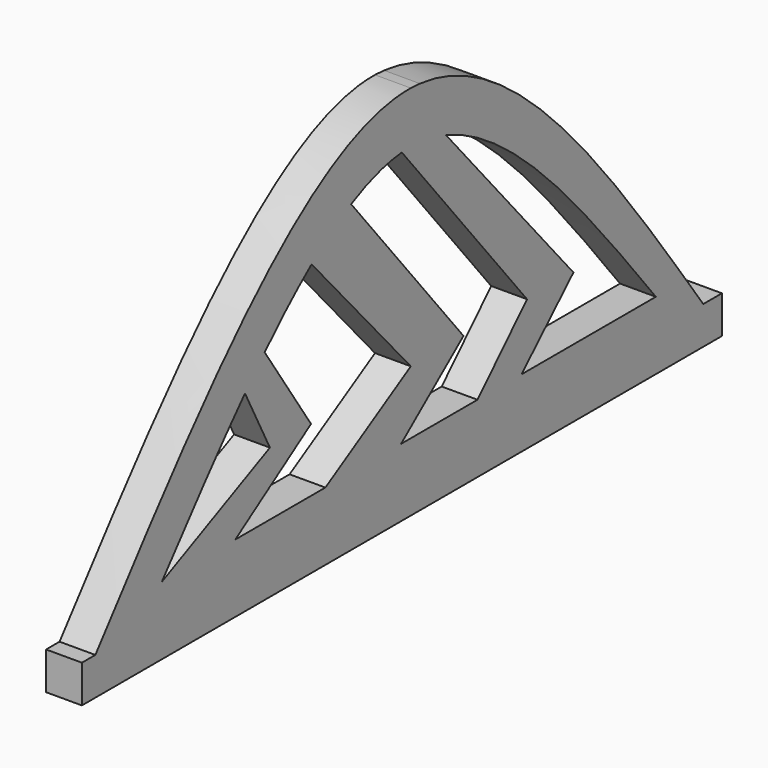
from build123d import *

# Parameters (mm, degrees)
F1_DEPTH = 7.62


with BuildPart() as f1:
    # F0 (on Right) → F1 (new body)
    with BuildSketch(Plane.YZ):
        with BuildLine():
            Line((-83.8999077678, 0), (-76.0438218713, 0))
            Line((-76.0438218713, 0), (-68.3361637849, 0))
            Line((-68.3361637849, 0), (-65.6663442796, 0))
            Line((-65.6663442796, 0), (-59.0906857838, 0))
            Line((-59.0906857838, 0), (-56.6208846061, 0))
            Line((-56.6208846061, 0), (-50.1111261547, 0))
            Line((-50.1111261547, 0), (-47.2127646201, 0))
            Line((-47.2127646201, 0), (-40.9584082663, 0))
            Line((-40.9584082663, 0), (-38.0600504577, 0))
            Line((-38.0600504577, 0), (-31.6531471908, 0))
            Line((-31.6531471908, 0), (-28.9073325694, 0))
            Line((-28.9073325694, 0), (-22.5004293025, 0))
            Line((-22.5004293025, 0), (-19.9071597308, 0))
            Line((-19.9071597308, 0), (-13.4495065357, 0))
            Line((-13.4495065357, 0), (-10.754442774, 0))
            Line((-10.754442774, 0), (-4.1949953884, 0))
            Line((-4.1949953884, 0), (-1.6017258168, 0))
            Line((-1.6017258168, 0), (4.8051769845, 0))
            Line((4.8051769845, 0), (7.3984456249, 0))
            Line((7.3984456249, 0), (13.8053493574, 0))
            Line((13.8053493574, 0), (16.7037080973, 0))
            Line((16.7037080973, 0), (23.1106095016, 0))
            Line((23.1106095016, 0), (25.7038809359, 0))
            Line((25.7038809359, 0), (32.1107842028, 0))
            Line((32.1107842028, 0), (34.5515049994, 0))
            Line((34.5515049994, 0), (40.958404541, 0))
            Line((40.958404541, 0), (43.7042228877, 0))
            Line((43.7042228877, 0), (50.1111261552, 0))
            Line((50.1111261552, 0), (52.7043938637, 0))
            Line((52.7043938637, 0), (59.263844043, 0))
            Line((59.263844043, 0), (61.8571154775, 0))
            Line((61.8571154775, 0), (72.8403702378, 0))
            Line((72.8403702378, 0), (77.7980908751, 0))
            add(Edge.make_bspline(
                [(2.4155534392, 71.935541455), (28.1982811761, 69.4119022605), (52.9981860256, 34.7059511303), (77.7980908751, 0)],
                knots=[0.5202204491, 0.5202204491, 0.5202204491, 0.5202204491, 1, 1, 1, 1], degree=3))
            add(Edge.make_bspline(
                [(2.4155534392, 71.935541455), (23.457256807, 69.5741418959), (44.3202320999, 38.0280369375), (65.1832073927, 6.4819319791)],
                knots=[0.5194057291, 0.5194057291, 0.5194057291, 0.5194057291, 1, 1, 1, 1], degree=3))
            Line((65.1832073927, 6.4819319791), (29.4485222548, 6.4819319791))
            Line((29.4485222548, 6.4819319791), (17.7436252383, 6.4819319791))
            Line((17.7436252383, 6.4819319791), (-2.5848655496, 6.4819319791))
            Line((-2.5848655496, 6.4819319791), (-22.7159410715, 6.4819319791))
            Line((-22.7159410715, 6.4819319791), (-46.667508781, 6.4819319791))
            Line((-46.667508781, 6.4819319791), (-66.2550926208, 6.4819319791))
            add(Edge.make_bspline(
                [(-66.2550926208, 6.4819319791), (-44.7386888592, 38.3814174671), (-23.2222850975, 70.2809029552), (-1.8906832982, 72.0038712376)],
                knots=[0, 0, 0, 0, 0.4866401258, 0.4866401258, 0.4866401258, 0.4866401258], degree=3))
            add(Edge.make_bspline(
                [(-1.8906832982, 72.0038712376), (-1.2602925513, 72.0547883357), (-0.6300631821, 72.0793517198), (2.66e-08, 72.0767825841)],
                knots=[0.4866401258, 0.4866401258, 0.4866401258, 0.4866401258, 0.5010212977, 0.5010212977, 0.5010212977, 0.5010212977], degree=3))
            add(Edge.make_bspline(
                [(-83.8999077678, 0), (-55.5586168349, 36.2935873023), (-27.217325902, 72.5871746046), (0, 72.0767825842)],
                knots=[0, 0, 0, 0, 0.505255101, 0.505255101, 0.505255101, 0.505255101], degree=3))
        make_face()
        Polygon((-68.3361637849, 0), (-76.0438218713, 0), (-83.8999077678, 0), (-87.4847173691, 0), (-87.4847173691, -8.0094942823), (82.7558115125, -8.0094942823), (82.7558115125, 0), (77.7980908751, 0), (72.8403702378, 0), (61.8571154775, 0), (59.263844043, 0), (52.7043938637, 0), (50.1111261552, 0), (43.7042228877, 0), (40.958404541, 0), (34.5515049994, 0), (32.1107842028, 0), (25.7038809359, 0), (23.1106095016, 0), (16.7037080973, 0), (13.8053493574, 0), (7.3984456249, 0), (4.8051769845, 0), (-1.6017258168, 0), (-4.1949953884, 0), (-10.754442774, 0), (-13.4495065357, 0), (-19.9071597308, 0), (-22.5004293025, 0), (-28.9073325694, 0), (-31.6531471908, 0), (-38.0600504577, 0), (-40.9584082663, 0), (-47.2127646201, 0), (-50.1111261547, 0), (-56.6208846061, 0), (-59.0906857838, 0), (-65.6663442796, 0), align=None)
        with BuildLine():
            add(Edge.make_bspline(
                [(0, 72.0767825842), (0.8061606012, 72.0616650837), (1.6113351386, 72.0142591471), (2.4155534392, 71.935541455)],
                knots=[0.505255101, 0.505255101, 0.505255101, 0.505255101, 0.5202204491, 0.5202204491, 0.5202204491, 0.5202204491], degree=3))
            add(Edge.make_bspline(
                [(-1.8906832982, 72.0038712376), (-1.2602925513, 72.0547883357), (-0.6300631821, 72.0793517198), (2.66e-08, 72.0767825841)],
                knots=[0.4866401258, 0.4866401258, 0.4866401258, 0.4866401258, 0.5010212977, 0.5010212977, 0.5010212977, 0.5010212977], degree=3))
            add(Edge.make_bspline(
                [(-66.2550926208, 6.4819319791), (-44.7386888592, 38.3814174671), (-23.2222850975, 70.2809029552), (-1.8906832982, 72.0038712376)],
                knots=[0, 0, 0, 0, 0.4866401258, 0.4866401258, 0.4866401258, 0.4866401258], degree=3))
            add(Edge.make_bspline(
                [(-66.2550926208, 6.4819319791), (-58.870002531, 15.6014280008), (-51.4849124411, 24.7209240225), (-44.1068523116, 32.8232360474)],
                knots=[0, 0, 0, 0, 0.1671216862, 0.1671216862, 0.1671216862, 0.1671216862], degree=3))
            add(Edge.make_bspline(
                [(-44.1068523116, 32.8232360474), (-42.3619029204, 34.7394747588), (-40.6173467479, 36.5988175914), (-38.8732767924, 38.3878083756)],
                knots=[0.1671216862, 0.1671216862, 0.1671216862, 0.1671216862, 0.2066468296, 0.2066468296, 0.2066468296, 0.2066468296], degree=3))
            add(Edge.make_bspline(
                [(-38.8732767924, 38.3878083756), (-34.7114395699, 42.6568392208), (-30.5523710257, 46.5252625196), (-26.3973348433, 49.8102324575)],
                knots=[0.2066468296, 0.2066468296, 0.2066468296, 0.2066468296, 0.3009648428, 0.3009648428, 0.3009648428, 0.3009648428], degree=3))
            add(Edge.make_bspline(
                [(-26.3973348433, 49.8102324575), (-22.8832827761, 52.5884406113), (-19.3721149148, 54.9493251989), (-15.8645956908, 56.7822785692)],
                knots=[0.3009648428, 0.3009648428, 0.3009648428, 0.3009648428, 0.3807327183, 0.3807327183, 0.3807327183, 0.3807327183], degree=3))
            add(Edge.make_bspline(
                [(-15.8645956908, 56.7822785692), (-11.3638797078, 59.1342549956), (-6.8691712251, 60.6169899499), (-2.3820852822, 60.9967989829)],
                knots=[0.3807327183, 0.3807327183, 0.3807327183, 0.3807327183, 0.4830878387, 0.4830878387, 0.4830878387, 0.4830878387], degree=3))
            add(Edge.make_bspline(
                [(-2.3820852822, 60.9967989829), (-1.5878150287, 61.0640299254), (2.3324808206, 61.2253407539), (6.2467363494, 60.5126612784), (9.3648919901, 59.4680160873)],
                knots=[0.4830878387, 0.4830878387, 0.4830878387, 0.4830878387, 0.5012059734, 0.5725407835, 0.5725407835, 0.5725407835, 0.5725407835], degree=3))
            add(Edge.make_bspline(
                [(9.3648919901, 59.4680160873), (28.0498000323, 53.2081940706), (46.6165037125, 29.8450630249), (65.1832073927, 6.4819319791)],
                knots=[0.5725407835, 0.5725407835, 0.5725407835, 0.5725407835, 1, 1, 1, 1], degree=3))
            add(Edge.make_bspline(
                [(2.4155534392, 71.935541455), (23.457256807, 69.5741418959), (44.3202320999, 38.0280369375), (65.1832073927, 6.4819319791)],
                knots=[0.5194057291, 0.5194057291, 0.5194057291, 0.5194057291, 1, 1, 1, 1], degree=3))
        make_face()
        with BuildLine():
            Line((-37.4757476613, 19.9564792332), (-66.2550926208, 6.4819319791))
            Line((-66.2550926208, 6.4819319791), (-46.667508781, 6.4819319791))
            Line((-46.667508781, 6.4819319791), (-26.5364367513, 19.9564792332))
            Line((-26.5364367513, 19.9564792332), (-38.8732767924, 38.3878083756))
            add(Edge.make_bspline(
                [(-44.1068523116, 32.8232360474), (-42.3619029204, 34.7394747588), (-40.6173467479, 36.5988175914), (-38.8732767924, 38.3878083756)],
                knots=[0.1671216862, 0.1671216862, 0.1671216862, 0.1671216862, 0.2066468296, 0.2066468296, 0.2066468296, 0.2066468296], degree=3))
            Line((-44.1068523116, 32.8232360474), (-37.4757476613, 19.9564792332))
        make_face()
        with BuildLine():
            Line((17.7436252383, 6.4819319791), (29.4485222548, 6.4819319791))
            Line((29.4485222548, 6.4819319791), (43.261088431, 19.9564792332))
            Line((43.261088431, 19.9564792332), (9.3648919901, 59.4680160873))
            add(Edge.make_bspline(
                [(-2.3820852822, 60.9967989829), (-1.5878150287, 61.0640299254), (2.3324808206, 61.2253407539), (6.2467363494, 60.5126612784), (9.3648919901, 59.4680160873)],
                knots=[0.4830878387, 0.4830878387, 0.4830878387, 0.4830878387, 0.5012059734, 0.5725407835, 0.5725407835, 0.5725407835, 0.5725407835], degree=3))
            Line((-2.3820852822, 60.9967989829), (30.9179425241, 19.9564792332))
            Line((30.9179425241, 19.9564792332), (17.7436252383, 6.4819319791))
        make_face()
        with BuildLine():
            Line((0, 19.9564792332), (-22.7159410715, 6.4819319791))
            Line((-22.7159410715, 6.4819319791), (-2.5848655496, 6.4819319791))
            Line((-2.5848655496, 6.4819319791), (14.0195973219, 19.9564792332))
            Line((14.0195973219, 19.9564792332), (-15.8645956908, 56.7822785692))
            add(Edge.make_bspline(
                [(-26.3973348433, 49.8102324575), (-22.8832827761, 52.5884406113), (-19.3721149148, 54.9493251989), (-15.8645956908, 56.7822785692)],
                knots=[0.3009648428, 0.3009648428, 0.3009648428, 0.3009648428, 0.3807327183, 0.3807327183, 0.3807327183, 0.3807327183], degree=3))
            Line((-26.3973348433, 49.8102324575), (0, 19.9564792332))
        make_face()
    extrude(amount=F1_DEPTH)


solid = f1.part
